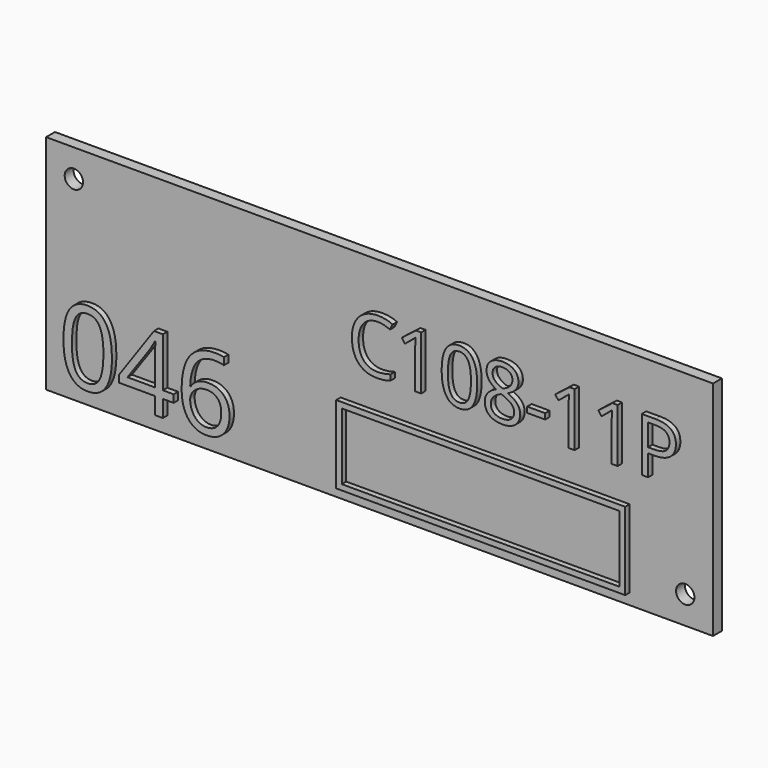
from build123d import *

# Parameters (mm, degrees)
F0_W         = 120
F0_H         = 40
F1_DEPTH     = 2
F3_D         = 3.3
F4_TEXT_SIZE = 13.553578992
F5_DEPTH     = 1
F6_TEXT_SIZE = 18.4837545126
F7_DEPTH     = 1
F8_W         = 52
F8_H         = 14
F8_W_2       = 49.99999962
F8_H_2       = 11.99999962
F9_DEPTH     = 1


# Not quite as in the source:
# - Text() gives the source's letters only with a copy of the font that has no kerning and outlines rounded to 1/6400 em; it was checked with that copy


with BuildPart() as f1:
    # F0 (on Front) → F1 (new body)
    with BuildSketch(Plane.XZ):
        Rectangle(F0_W, F0_H)
    extrude(amount=F1_DEPTH)

    # F3 (through all)
    with Locations(Plane.XZ.offset(2)):
        with Locations((-55, 15), (55, -15)):
            Hole(F3_D / 2)

    # F4 (on face) → F5 (join)
    with BuildSketch(Plane.XZ.offset(2)):
        with Locations((-5, 2)):
            Text('C108-11P', F4_TEXT_SIZE, font='Open Sans', text_align=(TextAlign.LEFT, TextAlign.BOTTOM))
    extrude(amount=F5_DEPTH)

    # F6 (on face) → F7 (join)
    with BuildSketch(Plane.XZ.offset(2)):
        with Locations((-57, -17)):
            Text('046', F6_TEXT_SIZE, font='Open Sans', text_align=(TextAlign.LEFT, TextAlign.BOTTOM))
    extrude(amount=F7_DEPTH)

    # F8 (on face) → F9 (join)
    with BuildSketch(Plane.XZ.offset(2)):
        with Locations((19, -11)):
            Rectangle(F8_W, F8_H)
        with Locations((19, -11)):
            Rectangle(F8_W_2, F8_H_2, mode=Mode.SUBTRACT)
    extrude(amount=F9_DEPTH)


solid = f1.part
